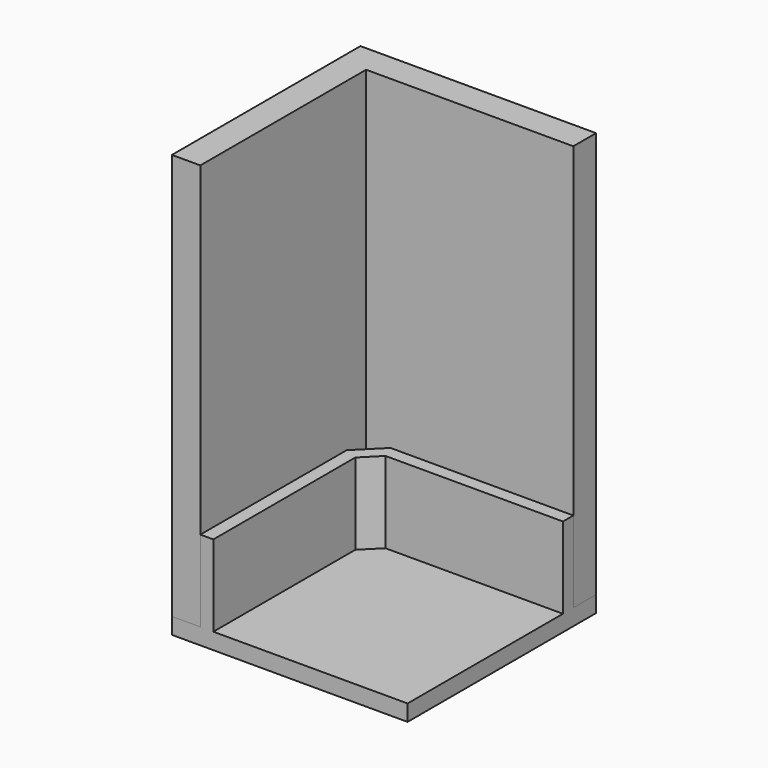
from build123d import *

# Parameters (mm, degrees)
F1_DEPTH = 50
F2_W     = 29
F2_H     = 29
F3_DEPTH = 2
F5_DEPTH = 10
F6_R     = 2


with BuildPart() as f1:
    # F0 (on Top) → F1 (new body)
    with BuildSketch(Plane.XY):
        Polygon((29, 0), (0, 0), (0, -29), (3.5, -29), (3.5, -3.5), (29, -3.5), align=None)
    extrude(amount=F1_DEPTH)


with BuildPart() as f3:
    # F2 (on Top) → F3 (new body)
    with BuildSketch(Plane.XY):
        with Locations((14.5, -14.5)):
            Rectangle(F2_W, F2_H)
    extrude(amount=-F3_DEPTH)

    # F4 (on face) → F5 (join)
    with BuildSketch(Plane.XY):
        Polygon((3.5, -29), (5.1, -29), (5.1, -7.1627416998), (7.1627416998, -5.1), (29, -5.1), (29, -3.5), (6.5, -3.5), (3.5, -6.5), align=None)
    extrude(amount=F5_DEPTH)

    # F6
    f6_edges = [f3.edges().sort_by_distance(p)[0] for p in [
        (0, 0, -1),
    ]]
    fillet(f6_edges, radius=F6_R)


solid = Compound([f1.part, f3.part])
